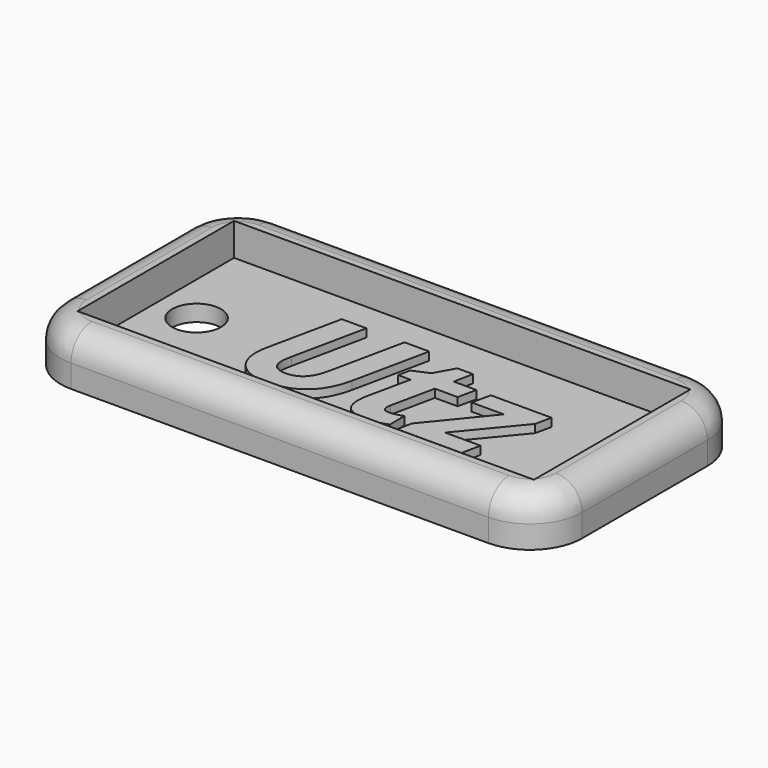
from build123d import *

# Parameters (mm, degrees)
F0_W         = 44.45
F0_H         = 19.05
F0_R         = 2.38125
F1_DEPTH     = 1.5875
F0_W_2       = 50.8
F0_H_2       = 25.4
F2_DEPTH     = 4.7625
F3_R         = 5.08
F4_T1_DEPTH  = 40.64
F4_T3_DEPTH  = 15.24
F4_T6_ANGLE  = 90
F4_T8_ANGLE  = 90
F4_T10_ANGLE = 90
F4_T12_ANGLE = 90
F5_TEXT_SIZE = 16.125041293
F6_DEPTH     = 0.79375


# Not quite as in the source:
# - a fillet or chamfer that OpenCascade refuses, or shapes differently, is made with other operations: its cross-section is extruded or revolved along the edge and cut away or added
# - Text() gives the source's letters only with a copy of the font that has no kerning and outlines rounded to 1/6400 em; it was checked with that copy


with BuildPart() as f1:
    # F0 (on Top) → F1 (new body)
    with BuildSketch(Plane.XY):
        with Locations((25.4, 12.7)):
            Rectangle(F0_W, F0_H)
        with Locations((7.14375, 12.7)):
            Circle(F0_R, mode=Mode.SUBTRACT)
    extrude(amount=F1_DEPTH)

    # F0 (on Top) → F2 (join)
    with BuildSketch(Plane.XY):
        with Locations((25.4, 12.7)):
            Rectangle(F0_W_2, F0_H_2)
        with Locations((25.4, 12.7)):
            Rectangle(F0_W, F0_H, mode=Mode.SUBTRACT)
    extrude(amount=F2_DEPTH)

    # F3
    f3_edges = [f1.edges().sort_by_distance(p)[0] for p in [
        (0, 0, 2.38125),
        (50.8, 0, 2.38125),
        (50.8, 25.4, 2.38125),
        (0, 25.4, 2.38125),
    ]]
    fillet(f3_edges, radius=F3_R)

    # F4: fillet of radius 2.54 on 8 edges, made by hand

    # F4_s2 → F4_t1 (cut)
    with BuildSketch(Plane.YZ.offset(5.08)):
        with BuildLine():
            ThreePointArc((25.4, 2.2225), (24.6560512242, 4.0185512242), (22.86, 4.7625))
            Line((22.86, 4.7625), (25.4, 4.7625))
            Line((25.4, 4.7625), (25.4, 2.2225))
        make_face()
        with BuildLine():
            ThreePointArc((0, 2.2225), (0.7439487758, 4.0185512242), (2.54, 4.7625))
            Line((2.54, 4.7625), (0, 4.7625))
            Line((0, 4.7625), (0, 2.2225))
        make_face()
    extrude(amount=F4_T1_DEPTH, mode=Mode.SUBTRACT)

    # F4_s4 → F4_t3 (cut)
    with BuildSketch(Plane.XZ.offset(-20.32)):
        with BuildLine():
            ThreePointArc((0, 2.2225), (0.7439487758, 4.0185512242), (2.54, 4.7625))
            Line((2.54, 4.7625), (0, 4.7625))
            Line((0, 4.7625), (0, 2.2225))
        make_face()
        with BuildLine():
            ThreePointArc((50.8, 2.2225), (50.0560512242, 4.0185512242), (48.26, 4.7625))
            Line((48.26, 4.7625), (50.8, 4.7625))
            Line((50.8, 4.7625), (50.8, 2.2225))
        make_face()
    extrude(amount=F4_T3_DEPTH, mode=Mode.SUBTRACT)

    # F4_s5 → F4_t6 (revolve, cut)
    with BuildSketch(Plane.XZ.offset(-20.32)):
        with BuildLine():
            ThreePointArc((0, 2.2225), (0.7439487758, 4.0185512242), (2.54, 4.7625))
            Line((2.54, 4.7625), (0, 4.7625))
            Line((0, 4.7625), (0, 2.2225))
        make_face()
    revolve(axis=Axis((5.08, 20.32, 4.7625), (0, 0, -1)), revolution_arc=F4_T6_ANGLE, mode=Mode.SUBTRACT)

    # F4_s7 → F4_t8 (revolve, cut)
    with BuildSketch(Plane.XZ.offset(-5.08)):
        with BuildLine():
            ThreePointArc((0, 2.2225), (0.7439487758, 4.0185512242), (2.54, 4.7625))
            Line((2.54, 4.7625), (0, 4.7625))
            Line((0, 4.7625), (0, 2.2225))
        make_face()
    revolve(axis=Axis((5.08, 5.08, 4.7625), (0, 0, 1)), revolution_arc=F4_T8_ANGLE, mode=Mode.SUBTRACT)

    # F4_s9 → F4_t10 (revolve, cut)
    with BuildSketch(Plane.XZ.offset(-20.32)):
        with BuildLine():
            ThreePointArc((50.8, 2.2225), (50.0560512242, 4.0185512242), (48.26, 4.7625))
            Line((48.26, 4.7625), (50.8, 4.7625))
            Line((50.8, 4.7625), (50.8, 2.2225))
        make_face()
    revolve(axis=Axis((45.72, 20.32, 4.7625), (0, 0, 1)), revolution_arc=F4_T10_ANGLE, mode=Mode.SUBTRACT)

    # F4_s11 → F4_t12 (revolve, cut)
    with BuildSketch(Plane.YZ.offset(45.72)):
        with BuildLine():
            ThreePointArc((0, 2.2225), (0.7439487758, 4.0185512242), (2.54, 4.7625))
            Line((2.54, 4.7625), (0, 4.7625))
            Line((0, 4.7625), (0, 2.2225))
        make_face()
    revolve(axis=Axis((45.72, 5.08, 4.7625), (0, 0, 1)), revolution_arc=F4_T12_ANGLE, mode=Mode.SUBTRACT)

    # F5 (on face) → F6 (join)
    with BuildSketch(Plane.XY.offset(1.5875)):
        with Locations((14.0604376793, 6.756877061)):
            Text('Utz', F5_TEXT_SIZE, font='Open Sans', font_style=FontStyle.BOLDITALIC, text_align=(TextAlign.LEFT, TextAlign.BOTTOM))
    extrude(amount=F6_DEPTH)


solid = f1.part
